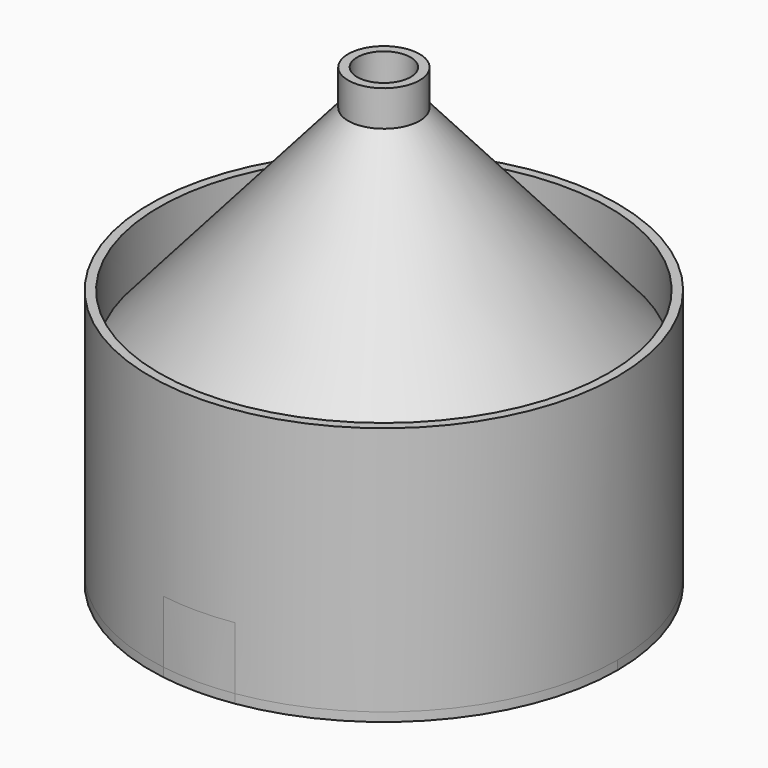
from build123d import *
from build123d import SkipClean  # not in build123d's __all__

# Parameters (mm, degrees)
F0_R      = 79.375
F0_R_2    = 76.2
F1_DEPTH  = 25.4
F4_R      = 79.375
F3_R      = 12.7
F7_R      = 9.525
F6_R      = 76.2
F9_R      = 12.7
F9_R_2    = 9.525
F10_DEPTH = 12.7
F11_R     = 83.185
F11_R_2   = 80.01
F12_DEPTH = 44.45
F14_DEPTH = 3.175
F15_R     = 83.185
F15_R_2   = 80.01
F16_DEPTH = 3.175
F17_R     = 2.54
F17_R_2   = 3.175
F18_DEPTH = 161.926
F20_DEPTH = 25.4


with BuildPart() as f1:
    # F0 (on Top) → F1 (new body)
    with BuildSketch(Plane.XY):
        Circle(F0_R)
        Circle(F0_R_2, mode=Mode.SUBTRACT)
    extrude(amount=F1_DEPTH)

    # F4 (on face) → F5 section 0
    with BuildSketch(Plane.XY.offset(25.4)):
        Circle(F4_R)
    # F3 (on offset) → F5 section 1
    with BuildSketch(Plane.XY.offset(101.6)):
        Circle(F3_R)
    loft()

    # F7 (on face) → F8 section 0
    with BuildSketch(Plane.XY.offset(101.6)):
        Circle(F7_R)
    # F6 (on face) → F8 section 1
    with BuildSketch(Plane(origin=(0, 0, 25.4), x_dir=(1, 0, 0), z_dir=(0, 0, -1))):
        Circle(F6_R)
    loft(mode=Mode.SUBTRACT)

    # F9 (on face) → F10 (join)
    with BuildSketch(Plane.XY.offset(101.6)):
        Circle(F9_R)
        Circle(F9_R_2, mode=Mode.SUBTRACT)
    extrude(amount=F10_DEPTH)


with BuildPart() as f12:
    # F11 (on face) → F12 (new body, symmetric)
    with BuildSketch(Plane(origin=(0, 0, 0), x_dir=(1, 0, 0), z_dir=(0, 0, -1))):
        Circle(F11_R)
        Circle(F11_R_2, mode=Mode.SUBTRACT)
    extrude(amount=F12_DEPTH, both=True)

    # F13 (on face) → F14 (join)
    with BuildSketch(Plane(origin=(0, 0, -44.45), x_dir=(1, 0, 0), z_dir=(0, 0, -1))):
        Polygon((-12.7, 104.3956334236), (-12.7, 78.9956334236), (-12.7, -78.9956334236), (-12.7, -104.3956334236), (12.7, -104.3956334236), (12.7, -78.9956334236), (12.7, 78.9956334236), (12.7, 104.3956334236), align=None)
    extrude(amount=F14_DEPTH)

    # F15 (on face) → F16 (join)
    with BuildSketch(Plane(origin=(0, 0, -44.45), x_dir=(1, 0, 0), z_dir=(0, 0, -1))):
        Circle(F15_R)
        Circle(F15_R_2, mode=Mode.SUBTRACT)
    extrude(amount=F16_DEPTH)

    # F17 (on face) → F18 (cut, through all)
    with BuildSketch(Plane(origin=(0, 0, -47.625), x_dir=(1, 0, 0), z_dir=(0, 0, -1))):
        with Locations((0, 14.2875)):
            Circle(F17_R)
        with Locations((0, -14.2875)):
            Circle(F17_R)
        with Locations((0, -41.91)):
            Circle(F17_R_2)
    extrude(amount=-F18_DEPTH, mode=Mode.SUBTRACT)

    # F19 (on face) → F20 (cut)
    with BuildSketch(Plane(origin=(0, 0, -47.625), x_dir=(1, 0, 0), z_dir=(0, 0, -1))):
        with BuildLine():
            Line((12.7, 104.3956334236), (-12.7, 104.3956334236))
            Line((-12.7, 104.3956334236), (-12.7, 82.2098183005))
            ThreePointArc((-12.7, 82.2098183005), (0, 83.185), (12.7, 82.2098183005))
            Line((12.7, 82.2098183005), (12.7, 104.3956334236))
        make_face()
        with BuildLine():
            ThreePointArc((12.7, -82.2098183005), (0, -83.185), (-12.7, -82.2098183005))
            Line((-12.7, -82.2098183005), (-12.7, -104.3956334236))
            Line((-12.7, -104.3956334236), (12.7, -104.3956334236))
            Line((12.7, -104.3956334236), (12.7, -82.2098183005))
        make_face()
    with SkipClean():  # cleaning this boolean's faces spoils the solid; the shape is the same uncleaned
        extrude(amount=-F20_DEPTH, mode=Mode.SUBTRACT)


solid = Compound([f1.part, f12.part])
